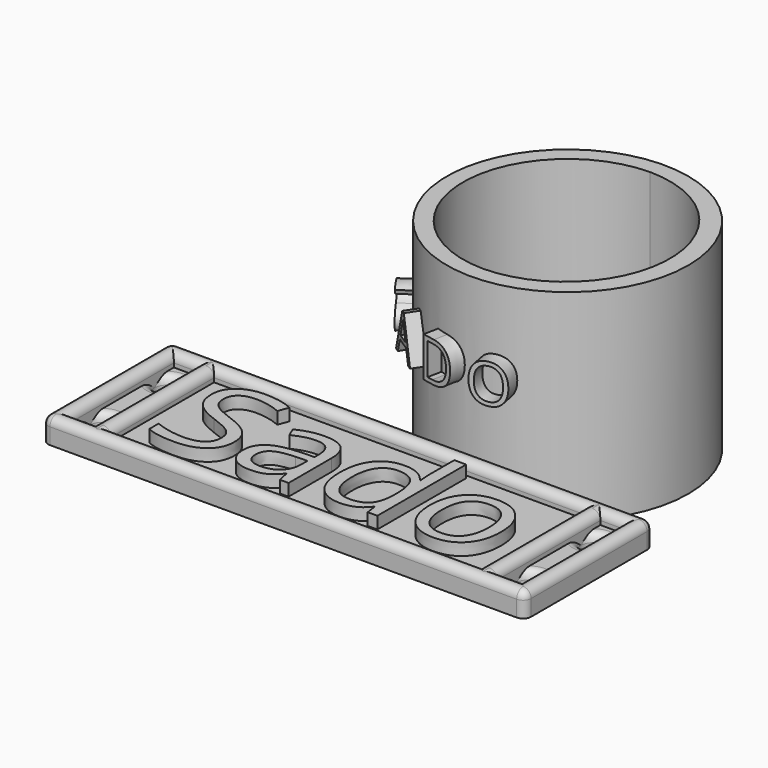
from build123d import *

# Parameters (mm, degrees)
F2_DEPTH       = 12.5
F3_TEXT_SIZE   = 7.2267029383
F4_DEPTH       = 2
F5_TEXT_SIZE   = 7.1017000462
F6_DEPTH       = 2
F7_TEXT_SIZE   = 6.9642465355
F8_DEPTH       = 2
F9_TEXT_SIZE   = 6.6435236173
F10_DEPTH      = 2
F1_R           = 15
F1_R_2         = 13
F11_DEPTH      = 12.5
F12_R          = 13
F13_DEPTH      = 70
F14_DEPTH      = 12.5
F15_W          = 46
F15_H          = 16
F15_TEXT_SIZE  = 18.1491124547
F16_DEPTH      = 3
F17_DEPTH      = 1.5
F18_T1_DEPTH   = 18
F18_T3_DEPTH   = 58
F18_T5_DEPTH   = 16
F18_T7_DEPTH   = 3
F18_T9_DEPTH   = 46
F18_T11_DEPTH  = 3
F18_T13_DEPTH  = 4.5
F18_S17_W      = 1.02
F18_S17_H      = 1.02
F18_T18_DEPTH  = 1.02
F18_S23_W      = 1.02
F18_S23_H      = 1.02
F18_T24_DEPTH  = 1.02
F18_S29_W      = 1.02
F18_S29_H      = 1.02
F18_T30_DEPTH  = 1.02
F18_S35_W      = 1.02
F18_S35_H      = 1.02
F18_T36_DEPTH  = 1.02
F18_T42_DEPTH  = 8
F18_T47_DEPTH  = 8
F18_T52_DEPTH  = 51
F18_T57_DEPTH  = 51
F18_T62_DEPTH  = 51
F18_T67_DEPTH  = 51
F18_T72_DEPTH  = 8
F18_T77_DEPTH  = 8
F18_T82_ANGLE  = 180
F18_T88_ANGLE  = 180
F18_T94_ANGLE  = 180
F18_T100_ANGLE = 180
F18_T106_ANGLE = 180
F18_T112_ANGLE = 180
F18_T118_ANGLE = 180
F18_T124_ANGLE = 180
F18_T131_DEPTH = 18.5
F18_T136_DEPTH = 5.5
F18_T144_DEPTH = 18.5
F18_T149_DEPTH = 5.5
F18_T157_DEPTH = 5.5
F18_T162_DEPTH = 18.5
F18_T170_DEPTH = 18.5
F18_T175_DEPTH = 5.5
F18_T183_DEPTH = 48.5
F18_T188_DEPTH = 18.5
F18_T196_DEPTH = 48.5
F18_T201_DEPTH = 18.5
F18_T209_DEPTH = 18.5
F18_T214_DEPTH = 48.5
F18_T222_DEPTH = 48.5
F18_T227_DEPTH = 18.5
F18_T235_DEPTH = 5.5
F18_T240_DEPTH = 18.5
F18_T248_DEPTH = 5.5
F18_T253_DEPTH = 18.5
F18_T261_DEPTH = 18.5
F18_T266_DEPTH = 5.5
F18_T274_DEPTH = 5.5
F18_T279_DEPTH = 18.5


# Not quite as in the source:
# - a fillet or chamfer that OpenCascade refuses, or shapes differently, is made with other operations: its cross-section is extruded or revolved along the edge and cut away or added
# - Text() gives the source's letters only with a copy of the font that has no kerning and outlines rounded to 1/6400 em; it was checked with that copy


with BuildPart() as f2:
    # F0 (on Top) → F2 (new body, symmetric)
    with BuildSketch(Plane.XY):
        Polygon((-5.7402514855, -13.8581929877), (0, -15), (5.7402514855, -13.8581929877), (10.6066017178, -10.6066017178), (13.8581929877, -5.7402514855), (15, 0), (13.8581929877, 5.7402514855), (10.6066017178, 10.6066017178), (5.7402514855, 13.8581929877), (0, 15), (-5.7402514855, 13.8581929877), (-10.6066017178, 10.6066017178), (-13.8581929877, 5.7402514855), (-15, 0), (-13.8581929877, -5.7402514855), (-10.6066017178, -10.6066017178), align=None)
    extrude(amount=F2_DEPTH, both=True)

    # F3 (on face) → F4 (join)
    with BuildSketch(Plane(origin=(-12.2323973527, -8.1734266016, 0), x_dir=(0.555570233, -0.8314696123, 0), z_dir=(-0.8314696123, -0.555570233, 0))):
        with Locations((-2.0443665109, 0)):
            Text('S', F3_TEXT_SIZE, font='Open Sans', text_align=(TextAlign.LEFT, TextAlign.BOTTOM))
    extrude(amount=F4_DEPTH)

    # F5 (on face) → F6 (join)
    with BuildSketch(Plane(origin=(-8.1734266016, -12.2323973527, 0), x_dir=(0.8314696123, -0.555570233, 0), z_dir=(-0.555570233, -0.8314696123, 0))):
        with Locations((-2.3712676484, 0)):
            Text('A', F5_TEXT_SIZE, font='Open Sans', text_align=(TextAlign.LEFT, TextAlign.BOTTOM))
    extrude(amount=F6_DEPTH)

    # F7 (on face) → F8 (join)
    with BuildSketch(Plane(origin=(-2.8701257427, -14.4290964938, 0), x_dir=(0.9807852804, -0.195090322, 0), z_dir=(-0.195090322, -0.9807852804, 0))):
        with Locations((-2.5102309883, 0)):
            Text('D', F7_TEXT_SIZE, font='Open Sans', text_align=(TextAlign.LEFT, TextAlign.BOTTOM))
    extrude(amount=F8_DEPTH)

    # F9 (on face) → F10 (join)
    with BuildSketch(Plane(origin=(2.8701257427, -14.4290964938, 0), x_dir=(0.9807852804, 0.195090322, 0), z_dir=(0.195090322, -0.9807852804, 0))):
        with Locations((-2.5762089062, 0)):
            Text('O', F9_TEXT_SIZE, font='Open Sans', text_align=(TextAlign.LEFT, TextAlign.BOTTOM))
    extrude(amount=F10_DEPTH)

    # F1 (on Top) → F11 (join, symmetric)
    with BuildSketch(Plane.XY):
        Circle(F1_R)
        Circle(F1_R_2, mode=Mode.SUBTRACT)
    extrude(amount=F11_DEPTH, both=True)

    # F12 (on face) → F13 (cut)
    with BuildSketch(Plane(origin=(0, 0, -12.5), x_dir=(1, 0, 0), z_dir=(0, 0, -1))):
        with Locations((-0.2790116705, 0)):
            Circle(F12_R)
    extrude(amount=-F13_DEPTH, mode=Mode.SUBTRACT)

    # F1 (on Top) → F14 (join, symmetric)
    with BuildSketch(Plane.XY):
        Circle(F1_R)
        Circle(F1_R_2, mode=Mode.SUBTRACT)
    extrude(amount=F14_DEPTH, both=True)


with BuildPart() as f16:
    # F15 (on Top) → F16 (new body)
    with BuildSketch(Plane.XY):
        Polygon((29.2240764946, -29.4431182742), (-20.7759235054, -29.4431182742), (-20.7759235054, -31.4431182742), (-20.7759235054, -34.4431193173), (-20.7759235054, -44.4431193173), (-20.7759235054, -47.4431182742), (-20.7759235054, -49.4431182742), (29.2240764946, -49.4431182742), (34.2240764946, -49.4431182742), (34.2240764946, -29.4431182742), align=None)
        with Locations((4.2240764946, -39.4431182742)):
            Rectangle(F15_W, F15_H, mode=Mode.SUBTRACT)
        Polygon((32.2240764946, -47.4431182742), (29.2240764946, -47.4431182742), (29.2240764946, -44.4431193173), (29.2240764946, -34.4431193173), (29.2240764946, -31.4431182742), (32.2240764946, -31.4431182742), (32.2240764946, -34.4431193173), (32.2240764946, -44.4431193173), align=None, mode=Mode.SUBTRACT)
        Polygon((-20.7759235054, -31.4431182742), (-20.7759235054, -29.4431182742), (-25.7759235054, -29.4431182742), (-25.7759235054, -49.4431182742), (-20.7759235054, -49.4431182742), (-20.7759235054, -47.4431182742), (-23.7759235054, -47.4431182742), (-23.7759235054, -44.4431193173), (-23.7759235054, -34.4431193173), (-23.7759235054, -31.4431182742), align=None)
        with Locations((-16.7070478201, -45.6872321665)):
            Text('Sado', F15_TEXT_SIZE, font='Open Sans', text_align=(TextAlign.LEFT, TextAlign.BOTTOM))
    extrude(amount=F16_DEPTH)

    # F15 (on Top) → F17 (join)
    with BuildSketch(Plane.XY):
        with Locations((4.2240764946, -39.4431182742)):
            Rectangle(F15_W, F15_H)
        with BuildLine():
            Line((1.8787776531, -45.6872321665), (0.786995107, -45.6872321665))
            Line((0.786995107, -45.6872321665), (0.4949078284, -44.3033623419))
            Line((0.4949078284, -44.3033623419), (0.4240128579, -44.3033623419))
            add(Edge.make_bspline(
                [(0.4240128579, -44.3033623419), (-0.3019516403, -45.2164895622), (-1.0236624403, -45.5411885272)],
                knots=[0, 0, 0, 1, 1, 1], degree=2))
            add(Edge.make_bspline(
                [(-1.0236624403, -45.5411885272), (-1.7453732402, -45.8658874923), (-2.8286483899, -45.8658874923)],
                knots=[0, 0, 0, 1, 1, 1], degree=2))
            add(Edge.make_bspline(
                [(-2.8286483899, -45.8658874923), (-4.2720699898, -45.8658874923), (-5.0916158491, -45.1200724023)],
                knots=[0, 0, 0, 1, 1, 1], degree=2))
            add(Edge.make_bspline(
                [(-5.0916158491, -45.1200724023), (-5.9111617084, -44.3742573124), (-5.9111617084, -43.001730683)],
                knots=[0, 0, 0, 1, 1, 1], degree=2))
            add(Edge.make_bspline(
                [(-5.9111617084, -43.001730683), (-5.9111617084, -40.0610073056), (-1.2065714642, -39.9192173645)],
                knots=[0, 0, 0, 1, 1, 1], degree=2))
            Line((-1.2065714642, -39.9192173645), (0.4410276508, -39.8653371869))
            Line((0.4410276508, -39.8653371869), (0.4410276508, -39.261312038))
            add(Edge.make_bspline(
                [(0.4410276508, -39.261312038), (0.4410276508, -38.1184851131), (-0.0495655452, -37.5740117395)],
                knots=[0, 0, 0, 1, 1, 1], degree=2))
            add(Edge.make_bspline(
                [(-0.0495655452, -37.5740117395), (-0.5401587413, -37.0295383659), (-1.6234338909, -37.0295383659)],
                knots=[0, 0, 0, 1, 1, 1], degree=2))
            add(Edge.make_bspline(
                [(-1.6234338909, -37.0295383659), (-2.8371557863, -37.0295383659), (-4.3684871497, -37.772517657)],
                knots=[0, 0, 0, 1, 1, 1], degree=2))
            Line((-4.3684871497, -37.772517657), (-4.8222149611, -36.646705525))
            add(Edge.make_bspline(
                [(-4.8222149611, -36.646705525), (-4.1047578593, -36.2582010865), (-3.2497645148, -36.0370087785)],
                knots=[0, 0, 0, 1, 1, 1], degree=2))
            add(Edge.make_bspline(
                [(-3.2497645148, -36.0370087785), (-2.3947711703, -35.8158164705), (-1.5326883287, -35.8158164705)],
                knots=[0, 0, 0, 1, 1, 1], degree=2))
            add(Edge.make_bspline(
                [(-1.5326883287, -35.8158164705), (0.2028205498, -35.8158164705), (1.0407991014, -36.5857358504)],
                knots=[0, 0, 0, 1, 1, 1], degree=2))
            add(Edge.make_bspline(
                [(1.0407991014, -36.5857358504), (1.8787776531, -37.3556552303), (1.8787776531, -39.0571345229)],
                knots=[0, 0, 0, 1, 1, 1], degree=2))
            Line((1.8787776531, -39.0571345229), (1.8787776531, -45.6872321665))
        make_face(mode=Mode.SUBTRACT)
        with BuildLine():
            add(Edge.make_bspline(
                [(23.2110742844, -37.1528956146), (24.4120350851, -38.5098253505), (24.4120350851, -40.8210013896)],
                knots=[0, 0, 0, 1, 1, 1], degree=2))
            add(Edge.make_bspline(
                [(24.4120350851, -40.8210013896), (24.4120350851, -43.1974008016), (23.2167458821, -44.531644147)],
                knots=[0, 0, 0, 1, 1, 1], degree=2))
            add(Edge.make_bspline(
                [(23.2167458821, -44.531644147), (22.021456679, -45.8658874923), (19.9116223561, -45.8658874923)],
                knots=[0, 0, 0, 1, 1, 1], degree=2))
            add(Edge.make_bspline(
                [(19.9116223561, -45.8658874923), (18.6071548984, -45.8658874923), (17.5976105181, -45.2533549469)],
                knots=[0, 0, 0, 1, 1, 1], degree=2))
            add(Edge.make_bspline(
                [(17.5976105181, -45.2533549469), (16.5880661379, -44.6408224016), (16.0379211666, -43.4979954767)],
                knots=[0, 0, 0, 1, 1, 1], degree=2))
            add(Edge.make_bspline(
                [(16.0379211666, -43.4979954767), (15.4877761953, -42.3551685518), (15.4877761953, -40.8210013896)],
                knots=[0, 0, 0, 1, 1, 1], degree=2))
            add(Edge.make_bspline(
                [(15.4877761953, -40.8210013896), (15.4877761953, -38.4474377764), (16.6759759013, -37.1217018275)],
                knots=[0, 0, 0, 1, 1, 1], degree=2))
            add(Edge.make_bspline(
                [(16.6759759013, -37.1217018275), (17.8641756073, -35.7959658787), (19.9740099302, -35.7959658787)],
                knots=[0, 0, 0, 1, 1, 1], degree=2))
            add(Edge.make_bspline(
                [(19.9740099302, -35.7959658787), (22.0101134837, -35.7959658787), (23.2110742844, -37.1528956146)],
                knots=[0, 0, 0, 1, 1, 1], degree=2))
        make_face(mode=Mode.SUBTRACT)
        with BuildLine():
            add(Edge.make_bspline(
                [(-8.3811424815, -40.0780220985), (-7.6154767998, -40.9117469519), (-7.6154767998, -42.2389008001)],
                knots=[0, 0, 0, 1, 1, 1], degree=2))
            add(Edge.make_bspline(
                [(-7.6154767998, -42.2389008001), (-7.6154767998, -43.9488874892), (-8.856138784, -44.9073874907)],
                knots=[0, 0, 0, 1, 1, 1], degree=2))
            add(Edge.make_bspline(
                [(-8.856138784, -44.9073874907), (-10.0968007682, -45.8658874923), (-12.223649884, -45.8658874923)],
                knots=[0, 0, 0, 1, 1, 1], degree=2))
            add(Edge.make_bspline(
                [(-12.223649884, -45.8658874923), (-14.5263185267, -45.8658874923), (-15.7683984103, -45.2703697398)],
                knots=[0, 0, 0, 1, 1, 1], degree=2))
            Line((-15.7683984103, -45.2703697398), (-15.7683984103, -43.8184407435))
            add(Edge.make_bspline(
                [(-15.7683984103, -43.8184407435), (-14.9687031428, -44.1530650043), (-14.030053733, -44.348735123)],
                knots=[0, 0, 0, 1, 1, 1], degree=2))
            add(Edge.make_bspline(
                [(-14.030053733, -44.348735123), (-13.0914043233, -44.5444052416), (-12.1697697064, -44.5444052416)],
                knots=[0, 0, 0, 1, 1, 1], degree=2))
            add(Edge.make_bspline(
                [(-12.1697697064, -44.5444052416), (-10.6639605324, -44.5444052416), (-9.9011306496, -43.9729917792)],
                knots=[0, 0, 0, 1, 1, 1], degree=2))
            add(Edge.make_bspline(
                [(-9.9011306496, -43.9729917792), (-9.1383007667, -43.4015783168), (-9.1383007667, -42.3806907412)],
                knots=[0, 0, 0, 1, 1, 1], degree=2))
            add(Edge.make_bspline(
                [(-9.1383007667, -42.3806907412), (-9.1383007667, -41.7086064206), (-9.4091195541, -41.2789828992)],
                knots=[0, 0, 0, 1, 1, 1], degree=2))
            add(Edge.make_bspline(
                [(-9.4091195541, -41.2789828992), (-9.6799383415, -40.8493593778), (-10.313739378, -40.4849592293)],
                knots=[0, 0, 0, 1, 1, 1], degree=2))
            add(Edge.make_bspline(
                [(-10.313739378, -40.4849592293), (-10.9475404145, -40.1205590808), (-12.2406646769, -39.6611596718)],
                knots=[0, 0, 0, 1, 1, 1], degree=2))
            add(Edge.make_bspline(
                [(-12.2406646769, -39.6611596718), (-14.0470685259, -39.0145975406), (-14.8226595035, -38.128410409)],
                knots=[0, 0, 0, 1, 1, 1], degree=2))
            add(Edge.make_bspline(
                [(-14.8226595035, -38.128410409), (-15.5982504811, -37.2422232774), (-15.5982504811, -35.8158164705)],
                knots=[0, 0, 0, 1, 1, 1], degree=2))
            add(Edge.make_bspline(
                [(-15.5982504811, -35.8158164705), (-15.5982504811, -34.3185146929), (-14.4738562485, -33.4323275614)],
                knots=[0, 0, 0, 1, 1, 1], degree=2))
            add(Edge.make_bspline(
                [(-14.4738562485, -33.4323275614), (-13.349462016, -32.5461404298), (-11.494849587, -32.5461404298)],
                knots=[0, 0, 0, 1, 1, 1], degree=2))
            add(Edge.make_bspline(
                [(-11.494849587, -32.5461404298), (-9.5636705899, -32.5461404298), (-7.9415936642, -33.255090135)],
                knots=[0, 0, 0, 1, 1, 1], degree=2))
            Line((-7.9415936642, -33.255090135), (-8.4123362685, -34.5652291904))
            add(Edge.make_bspline(
                [(-8.4123362685, -34.5652291904), (-10.0173984012, -33.8931448698), (-11.5317149717, -33.8931448698)],
                knots=[0, 0, 0, 1, 1, 1], degree=2))
            add(Edge.make_bspline(
                [(-11.5317149717, -33.8931448698), (-12.7284220742, -33.8931448698), (-13.4019242942, -34.4064244564)],
                knots=[0, 0, 0, 1, 1, 1], degree=2))
            add(Edge.make_bspline(
                [(-13.4019242942, -34.4064244564), (-14.0754265142, -34.919704043), (-14.0754265142, -35.8328312634)],
                knots=[0, 0, 0, 1, 1, 1], degree=2))
            add(Edge.make_bspline(
                [(-14.0754265142, -35.8328312634), (-14.0754265142, -36.504915584), (-13.8272941173, -36.9359570048)],
                knots=[0, 0, 0, 1, 1, 1], degree=2))
            add(Edge.make_bspline(
                [(-13.8272941173, -36.9359570048), (-13.5791617205, -37.3669984256), (-12.9893155657, -37.7257269764)],
                knots=[0, 0, 0, 1, 1, 1], degree=2))
            add(Edge.make_bspline(
                [(-12.9893155657, -37.7257269764), (-12.3994694109, -38.0844555273), (-11.1857475155, -38.5183327469)],
                knots=[0, 0, 0, 1, 1, 1], degree=2))
            add(Edge.make_bspline(
                [(-11.1857475155, -38.5183327469), (-9.1468081632, -39.2442972451), (-8.3811424815, -40.0780220985)],
                knots=[0, 0, 0, 1, 1, 1], degree=2))
        make_face(mode=Mode.SUBTRACT)
        with BuildLine():
            Line((11.7133279645, -45.6872321665), (11.5176578458, -44.3856005077))
            Line((11.5176578458, -44.3856005077), (11.4382554788, -44.3856005077))
            add(Edge.make_bspline(
                [(11.4382554788, -44.3856005077), (10.4202037021, -45.8658874923), (8.3897717462, -45.8658874923)],
                knots=[0, 0, 0, 1, 1, 1], degree=2))
            add(Edge.make_bspline(
                [(8.3897717462, -45.8658874923), (6.4841149385, -45.8658874923), (5.4249440788, -44.562837934)],
                knots=[0, 0, 0, 1, 1, 1], degree=2))
            add(Edge.make_bspline(
                [(5.4249440788, -44.562837934), (4.3657732191, -43.2597883757), (4.3657732191, -40.8578667743)],
                knots=[0, 0, 0, 1, 1, 1], degree=2))
            add(Edge.make_bspline(
                [(4.3657732191, -40.8578667743), (4.3657732191, -38.4559451729), (5.429197777, -37.1259555258)],
                knots=[0, 0, 0, 1, 1, 1], degree=2))
            add(Edge.make_bspline(
                [(5.429197777, -37.1259555258), (6.4926223349, -35.7959658787), (8.3897717462, -35.7959658787)],
                knots=[0, 0, 0, 1, 1, 1], degree=2))
            add(Edge.make_bspline(
                [(8.3897717462, -35.7959658787), (10.3663235245, -35.7959658787), (11.4212406859, -37.233715881)],
                knots=[0, 0, 0, 1, 1, 1], degree=2))
            Line((11.4212406859, -37.233715881), (11.5375084376, -37.233715881))
            Line((11.5375084376, -37.233715881), (11.4751208635, -36.5332735722))
            Line((11.4751208635, -36.5332735722), (11.4382554788, -35.8498460563))
            Line((11.4382554788, -35.8498460563), (11.4382554788, -31.8967424998))
            Line((11.4382554788, -31.8967424998), (12.910035067, -31.8967424998))
            Line((12.910035067, -31.8967424998), (12.910035067, -45.6872321665))
            Line((12.910035067, -45.6872321665), (11.7133279645, -45.6872321665))
        make_face(mode=Mode.SUBTRACT)
        with BuildLine():
            add(Edge.make_bspline(
                [(17.7493257551, -37.9951278644), (17.013435961, -38.9437025701), (17.013435961, -40.8210013896)],
                knots=[0, 0, 0, 1, 1, 1], degree=2))
            add(Edge.make_bspline(
                [(17.013435961, -40.8210013896), (17.013435961, -42.684121215), (17.7578331515, -43.6582181101)],
                knots=[0, 0, 0, 1, 1, 1], degree=2))
            add(Edge.make_bspline(
                [(17.7578331515, -43.6582181101), (18.5022303421, -44.6323150051), (19.945651942, -44.6323150051)],
                knots=[0, 0, 0, 1, 1, 1], degree=2))
            add(Edge.make_bspline(
                [(19.945651942, -44.6323150051), (21.3919093407, -44.6323150051), (22.1405602295, -43.6624718083)],
                knots=[0, 0, 0, 1, 1, 1], degree=2))
            add(Edge.make_bspline(
                [(22.1405602295, -43.6624718083), (22.8892111182, -42.6926286115), (22.8892111182, -40.8210013896)],
                knots=[0, 0, 0, 1, 1, 1], degree=2))
            add(Edge.make_bspline(
                [(22.8892111182, -40.8210013896), (22.8892111182, -38.9692247595), (22.1405602295, -38.0078889591)],
                knots=[0, 0, 0, 1, 1, 1], degree=2))
            add(Edge.make_bspline(
                [(22.1405602295, -38.0078889591), (21.3919093407, -37.0465531588), (19.9286371491, -37.0465531588)],
                knots=[0, 0, 0, 1, 1, 1], degree=2))
            add(Edge.make_bspline(
                [(19.9286371491, -37.0465531588), (18.4852155491, -37.0465531588), (17.7493257551, -37.9951278644)],
                knots=[0, 0, 0, 1, 1, 1], degree=2))
        make_face()
        with BuildLine():
            Line((29.2240764946, -34.4431193173), (29.2240764946, -44.4431193173))
            ThreePointArc((29.2240765542, -44.4431193173), (30.7240765542, -42.9431193173), (32.2240765542, -44.4431193173))
            Line((32.2240764946, -44.4431193173), (32.2240764946, -34.4431193173))
            ThreePointArc((32.2240765542, -34.4431193173), (30.7240765542, -35.9431193173), (29.2240765542, -34.4431193173))
        make_face()
        with BuildLine():
            Line((29.2240764946, -31.4431182742), (29.2240764946, -34.4431193173))
            ThreePointArc((29.2240765542, -34.4431193173), (30.7240765542, -32.9431193173), (32.2240765542, -34.4431193173))
            Line((32.2240764946, -34.4431193173), (32.2240764946, -31.4431182742))
            Line((32.2240764946, -31.4431182742), (29.2240764946, -31.4431182742))
        make_face()
        with BuildLine():
            Line((29.2240764946, -44.4431193173), (29.2240764946, -47.4431182742))
            Line((29.2240764946, -47.4431182742), (32.2240764946, -47.4431182742))
            Line((32.2240764946, -47.4431182742), (32.2240764946, -44.4431193173))
            ThreePointArc((32.2240765542, -44.4431193173), (30.7240765542, -45.9431193173), (29.2240765542, -44.4431193173))
        make_face()
        with BuildLine():
            add(Edge.make_bspline(
                [(6.5734426013, -43.6837402995), (7.2554522178, -44.6323150051), (8.5769344684, -44.6323150051)],
                knots=[0, 0, 0, 1, 1, 1], degree=2))
            add(Edge.make_bspline(
                [(8.5769344684, -44.6323150051), (10.0827436424, -44.6323150051), (10.7604995606, -43.8127691458)],
                knots=[0, 0, 0, 1, 1, 1], degree=2))
            add(Edge.make_bspline(
                [(10.7604995606, -43.8127691458), (11.4382554788, -42.9932232865), (11.4382554788, -41.1669688458)],
                knots=[0, 0, 0, 1, 1, 1], degree=2))
            Line((11.4382554788, -41.1669688458), (11.4382554788, -40.8578667743))
            add(Edge.make_bspline(
                [(11.4382554788, -40.8578667743), (11.4382554788, -38.7934052326), (10.7519921641, -37.9114717992)],
                knots=[0, 0, 0, 1, 1, 1], degree=2))
            add(Edge.make_bspline(
                [(10.7519921641, -37.9114717992), (10.0657288494, -37.0295383659), (8.5599196755, -37.0295383659)],
                knots=[0, 0, 0, 1, 1, 1], degree=2))
            add(Edge.make_bspline(
                [(8.5599196755, -37.0295383659), (7.2639596142, -37.0295383659), (6.5776962995, -38.0348290479)],
                knots=[0, 0, 0, 1, 1, 1], degree=2))
            add(Edge.make_bspline(
                [(6.5776962995, -38.0348290479), (5.8914329849, -39.04011973), (5.8914329849, -40.8748815672)],
                knots=[0, 0, 0, 1, 1, 1], degree=2))
            add(Edge.make_bspline(
                [(5.8914329849, -40.8748815672), (5.8914329849, -42.7351655938), (6.5734426013, -43.6837402995)],
                knots=[0, 0, 0, 1, 1, 1], degree=2))
        make_face()
        with BuildLine():
            add(Edge.make_bspline(
                [(-3.8864013501, -44.2338852707), (-3.4043155505, -44.649329798), (-2.5365611113, -44.649329798)],
                knots=[0, 0, 0, 1, 1, 1], degree=2))
            add(Edge.make_bspline(
                [(-2.5365611113, -44.649329798), (-1.1611986831, -44.649329798), (-0.3771003091, -43.896425211)],
                knots=[0, 0, 0, 1, 1, 1], degree=2))
            add(Edge.make_bspline(
                [(-0.3771003091, -43.896425211), (0.4069980649, -43.143520624), (0.4069980649, -41.7880087876)],
                knots=[0, 0, 0, 1, 1, 1], degree=2))
            Line((0.4069980649, -41.7880087876), (0.4069980649, -40.9117469519))
            Line((0.4069980649, -40.9117469519), (-1.0647815232, -40.9712987271))
            add(Edge.make_bspline(
                [(-1.0647815232, -40.9712987271), (-2.8201409934, -41.0336863012), (-3.5943140716, -41.5171900002)],
                knots=[0, 0, 0, 1, 1, 1], degree=2))
            add(Edge.make_bspline(
                [(-3.5943140716, -41.5171900002), (-4.3684871497, -42.0006936992), (-4.3684871497, -43.0187454759)],
                knots=[0, 0, 0, 1, 1, 1], degree=2))
            add(Edge.make_bspline(
                [(-4.3684871497, -43.0187454759), (-4.3684871497, -43.8184407435), (-3.8864013501, -44.2338852707)],
                knots=[0, 0, 0, 1, 1, 1], degree=2))
        make_face()
        with BuildLine():
            Line((-20.7759235054, -44.4431193173), (-20.7759235054, -34.4431193173))
            ThreePointArc((-20.775923565, -34.4431193173), (-22.275923565, -35.9431193173), (-23.775923565, -34.4431193173))
            Line((-23.7759235054, -34.4431193173), (-23.7759235054, -44.4431193173))
            ThreePointArc((-23.775923565, -44.4431193173), (-22.275923565, -42.9431193173), (-20.775923565, -44.4431193173))
        make_face()
        with BuildLine():
            Line((-20.7759235054, -34.4431193173), (-20.7759235054, -31.4431182742))
            Line((-20.7759235054, -31.4431182742), (-23.7759235054, -31.4431182742))
            Line((-23.7759235054, -31.4431182742), (-23.7759235054, -34.4431193173))
            ThreePointArc((-23.775923565, -34.4431193173), (-22.275923565, -32.9431193173), (-20.775923565, -34.4431193173))
        make_face()
        with BuildLine():
            Line((-20.7759235054, -47.4431182742), (-20.7759235054, -44.4431193173))
            ThreePointArc((-20.775923565, -44.4431193173), (-22.275923565, -45.9431193173), (-23.775923565, -44.4431193173))
            Line((-23.7759235054, -44.4431193173), (-23.7759235054, -47.4431182742))
            Line((-23.7759235054, -47.4431182742), (-20.7759235054, -47.4431182742))
        make_face()
    extrude(amount=F17_DEPTH)

    # F18: fillet of radius 1 on 28 edges, made by hand

    # F18_s2 → F18_t1 (cut)
    with BuildSketch(Plane.XZ.offset(30.4431182742)):
        with BuildLine():
            ThreePointArc((-25.7759235054, 2), (-25.4830302866, 2.7071067812), (-24.7759235054, 3))
            Line((-24.7759235054, 3), (-25.7759235054, 3))
            Line((-25.7759235054, 3), (-25.7759235054, 2))
        make_face()
        with BuildLine():
            ThreePointArc((33.2240764946, 3), (33.9311832758, 2.7071067812), (34.2240764946, 2))
            Line((34.2240764946, 2), (34.2240764946, 3))
            Line((34.2240764946, 3), (33.2240764946, 3))
        make_face()
    extrude(amount=F18_T1_DEPTH, mode=Mode.SUBTRACT)

    # F18_s4 → F18_t3 (cut)
    with BuildSketch(Plane.YZ.offset(-24.7759235054)):
        with BuildLine():
            ThreePointArc((-48.4431182742, 3), (-49.1502250554, 2.7071067812), (-49.4431182742, 2))
            Line((-49.4431182742, 2), (-49.4431182742, 3))
            Line((-49.4431182742, 3), (-48.4431182742, 3))
        make_face()
        with BuildLine():
            ThreePointArc((-30.4431182742, 3), (-29.736011493, 2.7071067812), (-29.4431182742, 2))
            Line((-29.4431182742, 2), (-29.4431182742, 3))
            Line((-29.4431182742, 3), (-30.4431182742, 3))
        make_face()
    extrude(amount=F18_T3_DEPTH, mode=Mode.SUBTRACT)

    # F18_s6 → F18_t5 (cut)
    with BuildSketch(Plane.XZ.offset(31.4431182742)):
        with BuildLine():
            ThreePointArc((-19.7759235054, 3), (-20.4830302866, 2.7071067812), (-20.7759235054, 2))
            Line((-20.7759235054, 2), (-20.7759235054, 3))
            Line((-20.7759235054, 3), (-19.7759235054, 3))
        make_face()
        with BuildLine():
            ThreePointArc((-24.7759235054, 3), (-24.0688167242, 2.7071067812), (-23.7759235054, 2))
            Line((-23.7759235054, 2), (-23.7759235054, 3))
            Line((-23.7759235054, 3), (-24.7759235054, 3))
        make_face()
        with BuildLine():
            ThreePointArc((-19.7759235054, 3), (-19.0688167242, 2.7071067812), (-18.7759235054, 2))
            Line((-18.7759235054, 2), (-18.7759235054, 3))
            Line((-18.7759235054, 3), (-19.7759235054, 3))
        make_face()
        with BuildLine():
            ThreePointArc((28.2240764946, 3), (27.5169697134, 2.7071067812), (27.2240764946, 2))
            Line((27.2240764946, 2), (27.2240764946, 3))
            Line((27.2240764946, 3), (28.2240764946, 3))
        make_face()
        with BuildLine():
            ThreePointArc((33.2240764946, 3), (32.5169697134, 2.7071067812), (32.2240764946, 2))
            Line((32.2240764946, 2), (32.2240764946, 3))
            Line((32.2240764946, 3), (33.2240764946, 3))
        make_face()
        with BuildLine():
            ThreePointArc((28.2240764946, 3), (28.9311832758, 2.7071067812), (29.2240764946, 2))
            Line((29.2240764946, 2), (29.2240764946, 3))
            Line((29.2240764946, 3), (28.2240764946, 3))
        make_face()
    extrude(amount=F18_T5_DEPTH, mode=Mode.SUBTRACT)

    # F18_s8 → F18_t7 (cut)
    with BuildSketch(Plane.YZ.offset(-23.7759235054)):
        with BuildLine():
            ThreePointArc((-48.4431182742, 3), (-47.736011493, 2.7071067812), (-47.4431182742, 2))
            Line((-47.4431182742, 2), (-47.4431182742, 3))
            Line((-47.4431182742, 3), (-48.4431182742, 3))
        make_face()
        with BuildLine():
            ThreePointArc((-30.4431182742, 3), (-31.1502250554, 2.7071067812), (-31.4431182742, 2))
            Line((-31.4431182742, 2), (-31.4431182742, 3))
            Line((-31.4431182742, 3), (-30.4431182742, 3))
        make_face()
    extrude(amount=F18_T7_DEPTH, mode=Mode.SUBTRACT)

    # F18_s10 → F18_t9 (cut)
    with BuildSketch(Plane.YZ.offset(-18.7759235054)):
        with BuildLine():
            ThreePointArc((-48.4431182742, 3), (-47.736011493, 2.7071067812), (-47.4431182742, 2))
            Line((-47.4431182742, 2), (-47.4431182742, 3))
            Line((-47.4431182742, 3), (-48.4431182742, 3))
        make_face()
        with BuildLine():
            ThreePointArc((-30.4431182742, 3), (-31.1502250554, 2.7071067812), (-31.4431182742, 2))
            Line((-31.4431182742, 2), (-31.4431182742, 3))
            Line((-31.4431182742, 3), (-30.4431182742, 3))
        make_face()
    extrude(amount=F18_T9_DEPTH, mode=Mode.SUBTRACT)

    # F18_s12 → F18_t11 (cut)
    with BuildSketch(Plane.YZ.offset(29.2240764946)):
        with BuildLine():
            ThreePointArc((-30.4431182742, 3), (-31.1502250554, 2.7071067812), (-31.4431182742, 2))
            Line((-31.4431182742, 2), (-31.4431182742, 3))
            Line((-31.4431182742, 3), (-30.4431182742, 3))
        make_face()
        with BuildLine():
            ThreePointArc((-48.4431182742, 3), (-47.736011493, 2.7071067812), (-47.4431182742, 2))
            Line((-47.4431182742, 2), (-47.4431182742, 3))
            Line((-47.4431182742, 3), (-48.4431182742, 3))
        make_face()
    extrude(amount=F18_T11_DEPTH, mode=Mode.SUBTRACT)

    # F18_s14 → F18_t13 (cut)
    with BuildSketch(Plane.XY.offset(-2.5)):
        with BuildLine():
            ThreePointArc((-25.7759235054, -48.4431182742), (-25.4830302866, -49.1502250554), (-24.7759235054, -49.4431182742))
            Line((-24.7759235054, -49.4431182742), (-25.7759235054, -49.4431182742))
            Line((-25.7759235054, -49.4431182742), (-25.7759235054, -48.4431182742))
        make_face()
        with BuildLine():
            ThreePointArc((-25.7759235054, -30.4431182742), (-25.4830302866, -29.736011493), (-24.7759235054, -29.4431182742))
            Line((-24.7759235054, -29.4431182742), (-25.7759235054, -29.4431182742))
            Line((-25.7759235054, -29.4431182742), (-25.7759235054, -30.4431182742))
        make_face()
        with BuildLine():
            ThreePointArc((34.2240764946, -30.4431182742), (33.9311832758, -29.736011493), (33.2240764946, -29.4431182742))
            Line((33.2240764946, -29.4431182742), (34.2240764946, -29.4431182742))
            Line((34.2240764946, -29.4431182742), (34.2240764946, -30.4431182742))
        make_face()
        with BuildLine():
            ThreePointArc((34.2240764946, -48.4431182742), (33.9311832758, -49.1502250554), (33.2240764946, -49.4431182742))
            Line((33.2240764946, -49.4431182742), (34.2240764946, -49.4431182742))
            Line((34.2240764946, -49.4431182742), (34.2240764946, -48.4431182742))
        make_face()
    extrude(amount=F18_T13_DEPTH, mode=Mode.SUBTRACT)


with BuildPart() as f18_tool16:
    # F18_s17 → F18_t18 (new body)
    with BuildSketch(Plane.YZ.offset(-24.7759235054)):
        with Locations((-29.9331182742, 2.51)):
            Rectangle(F18_S17_W, F18_S17_H)
    extrude(amount=-F18_T18_DEPTH)

    # F18_s19 → F18_t20 (revolve, cut)
    with BuildSketch(Plane(origin=(-24.7759235054, -30.4431182742, 2), x_dir=(0, -0.7071067812, -0.7071067812), z_dir=(0, 0.7071067812, -0.7071067812))):
        with BuildLine():
            ThreePointArc((0, -1), (1, 0), (0, 1))
            Line((0, 1), (0, -1))
        make_face()
    revolve(axis=Axis((-24.7759235054, -30.4431182742, 2), (-1, 0, 0)), mode=Mode.SUBTRACT)


with BuildPart() as f16_1:
    add(f16.part)

    # F18_t15: cut F18_tool16
    add(f18_tool16.part, mode=Mode.SUBTRACT)


with BuildPart() as f18_tool22:
    # F18_s23 → F18_t24 (new body)
    with BuildSketch(Plane.YZ.offset(-24.7759235054)):
        with Locations((-48.9531182742, 2.51)):
            Rectangle(F18_S23_W, F18_S23_H)
    extrude(amount=-F18_T24_DEPTH)

    # F18_s25 → F18_t26 (revolve, cut)
    with BuildSketch(Plane(origin=(-24.7759235054, -48.4431182742, 2), x_dir=(0, 0.7071067812, -0.7071067812), z_dir=(0, 0.7071067812, 0.7071067812))):
        with BuildLine():
            ThreePointArc((0, -1), (1, 0), (0, 1))
            Line((0, 1), (0, -1))
        make_face()
    revolve(axis=Axis((-24.7759235054, -48.4431182742, 2), (-1, 0, 0)), mode=Mode.SUBTRACT)


with BuildPart() as f16_2:
    add(f16_1.part)

    # F18_t21: cut F18_tool22
    add(f18_tool22.part, mode=Mode.SUBTRACT)


with BuildPart() as f18_tool28:
    # F18_s29 → F18_t30 (new body)
    with BuildSketch(Plane.YZ.offset(33.2240764946)):
        with Locations((-48.9531182742, 2.51)):
            Rectangle(F18_S29_W, F18_S29_H)
    extrude(amount=F18_T30_DEPTH)

    # F18_s31 → F18_t32 (revolve, cut)
    with BuildSketch(Plane(origin=(33.2240764946, -48.4431182742, 2), x_dir=(0, 0.7071067812, -0.7071067812), z_dir=(0, -0.7071067812, -0.7071067812))):
        with BuildLine():
            ThreePointArc((0, -1), (1, 0), (0, 1))
            Line((0, 1), (0, -1))
        make_face()
    revolve(axis=Axis((33.2240764946, -48.4431182742, 2), (1, 0, 0)), mode=Mode.SUBTRACT)


with BuildPart() as f16_3:
    add(f16_2.part)

    # F18_t27: cut F18_tool28
    add(f18_tool28.part, mode=Mode.SUBTRACT)


with BuildPart() as f18_tool34:
    # F18_s35 → F18_t36 (new body)
    with BuildSketch(Plane.YZ.offset(33.2240764946)):
        with Locations((-29.9331182742, 2.51)):
            Rectangle(F18_S35_W, F18_S35_H)
    extrude(amount=F18_T36_DEPTH)

    # F18_s37 → F18_t38 (revolve, cut)
    with BuildSketch(Plane(origin=(33.2240764946, -30.4431182742, 2), x_dir=(0, -0.7071067812, -0.7071067812), z_dir=(0, -0.7071067812, 0.7071067812))):
        with BuildLine():
            ThreePointArc((0, -1), (1, 0), (0, 1))
            Line((0, 1), (0, -1))
        make_face()
    revolve(axis=Axis((33.2240764946, -30.4431182742, 2), (1, 0, 0)), mode=Mode.SUBTRACT)


with BuildPart() as f16_4:
    add(f16_3.part)

    # F18_t33: cut F18_tool34
    add(f18_tool34.part, mode=Mode.SUBTRACT)


with BuildPart() as f18_tool40:
    # F18_s41 → F18_t42 (new body)
    with BuildSketch(Plane.YZ.offset(-18.2759235054)):
        with BuildLine():
            ThreePointArc((-48.4431182742, 3), (-47.736011493, 2.7071067812), (-47.4431182742, 2))
            Line((-47.4431182742, 2), (-47.4431182742, 3))
            Line((-47.4431182742, 3), (-48.4431182742, 3))
        make_face()
    extrude(amount=-F18_T42_DEPTH)

    split(bisect_by=Plane.YZ.offset(-18.7759235054), keep=Keep.TOP)


with BuildPart() as f16_5:
    add(f16_4.part)

    # F18_t39: cut F18_tool40
    add(f18_tool40.part, mode=Mode.SUBTRACT)


with BuildPart() as f18_tool45:
    # F18_s46 → F18_t47 (new body)
    with BuildSketch(Plane.YZ.offset(-26.2759235054)):
        with BuildLine():
            ThreePointArc((-30.4431182742, 3), (-31.1502250554, 2.7071067812), (-31.4431182742, 2))
            Line((-31.4431182742, 2), (-31.4431182742, 3))
            Line((-31.4431182742, 3), (-30.4431182742, 3))
        make_face()
    extrude(amount=F18_T47_DEPTH)

    split(bisect_by=Plane.YZ.offset(-18.7759235054), keep=Keep.TOP)


with BuildPart() as f16_6:
    add(f16_5.part)

    # F18_t44: cut F18_tool45
    add(f18_tool45.part, mode=Mode.SUBTRACT)


with BuildPart() as f18_tool50:
    # F18_s51 → F18_t52 (new body)
    with BuildSketch(Plane.YZ.offset(29.7240764946)):
        with BuildLine():
            ThreePointArc((-48.4431182742, 3), (-47.736011493, 2.7071067812), (-47.4431182742, 2))
            Line((-47.4431182742, 2), (-47.4431182742, 3))
            Line((-47.4431182742, 3), (-48.4431182742, 3))
        make_face()
    extrude(amount=-F18_T52_DEPTH)

    split(bisect_by=Plane.YZ.offset(29.2240764946), keep=Keep.TOP)


with BuildPart() as f16_7:
    add(f16_6.part)

    # F18_t49: cut F18_tool50
    add(f18_tool50.part, mode=Mode.SUBTRACT)


with BuildPart() as f18_tool55:
    # F18_s56 → F18_t57 (new body)
    with BuildSketch(Plane.YZ.offset(29.7240764946)):
        with BuildLine():
            ThreePointArc((-48.4431182742, 3), (-47.736011493, 2.7071067812), (-47.4431182742, 2))
            Line((-47.4431182742, 2), (-47.4431182742, 3))
            Line((-47.4431182742, 3), (-48.4431182742, 3))
        make_face()
    extrude(amount=-F18_T57_DEPTH)

    split(bisect_by=Plane.YZ.offset(-20.7759235054), keep=Keep.BOTTOM)


with BuildPart() as f16_8:
    add(f16_7.part)

    # F18_t54: cut F18_tool55
    add(f18_tool55.part, mode=Mode.SUBTRACT)


with BuildPart() as f18_tool60:
    # F18_s61 → F18_t62 (new body)
    with BuildSketch(Plane.YZ.offset(-21.2759235054)):
        with BuildLine():
            ThreePointArc((-30.4431182742, 3), (-31.1502250554, 2.7071067812), (-31.4431182742, 2))
            Line((-31.4431182742, 2), (-31.4431182742, 3))
            Line((-31.4431182742, 3), (-30.4431182742, 3))
        make_face()
    extrude(amount=F18_T62_DEPTH)

    split(bisect_by=Plane.YZ.offset(-20.7759235054), keep=Keep.BOTTOM)


with BuildPart() as f16_9:
    add(f16_8.part)

    # F18_t59: cut F18_tool60
    add(f18_tool60.part, mode=Mode.SUBTRACT)


with BuildPart() as f18_tool65:
    # F18_s66 → F18_t67 (new body)
    with BuildSketch(Plane.YZ.offset(-21.2759235054)):
        with BuildLine():
            ThreePointArc((-30.4431182742, 3), (-31.1502250554, 2.7071067812), (-31.4431182742, 2))
            Line((-31.4431182742, 2), (-31.4431182742, 3))
            Line((-31.4431182742, 3), (-30.4431182742, 3))
        make_face()
    extrude(amount=F18_T67_DEPTH)

    split(bisect_by=Plane.YZ.offset(29.2240764946), keep=Keep.TOP)


with BuildPart() as f16_10:
    add(f16_9.part)

    # F18_t64: cut F18_tool65
    add(f18_tool65.part, mode=Mode.SUBTRACT)


with BuildPart() as f18_tool70:
    # F18_s71 → F18_t72 (new body)
    with BuildSketch(Plane.YZ.offset(26.7240764946)):
        with BuildLine():
            ThreePointArc((-30.4431182742, 3), (-31.1502250554, 2.7071067812), (-31.4431182742, 2))
            Line((-31.4431182742, 2), (-31.4431182742, 3))
            Line((-31.4431182742, 3), (-30.4431182742, 3))
        make_face()
    extrude(amount=F18_T72_DEPTH)

    split(bisect_by=Plane.YZ.offset(27.2240764946), keep=Keep.BOTTOM)


with BuildPart() as f16_11:
    add(f16_10.part)

    # F18_t69: cut F18_tool70
    add(f18_tool70.part, mode=Mode.SUBTRACT)


with BuildPart() as f18_tool75:
    # F18_s76 → F18_t77 (new body)
    with BuildSketch(Plane.YZ.offset(34.7240764946)):
        with BuildLine():
            ThreePointArc((-48.4431182742, 3), (-47.736011493, 2.7071067812), (-47.4431182742, 2))
            Line((-47.4431182742, 2), (-47.4431182742, 3))
            Line((-47.4431182742, 3), (-48.4431182742, 3))
        make_face()
    extrude(amount=-F18_T77_DEPTH)

    split(bisect_by=Plane.YZ.offset(27.2240764946), keep=Keep.BOTTOM)


with BuildPart() as f16_12:
    add(f16_11.part)

    # F18_t74: cut F18_tool75
    add(f18_tool75.part, mode=Mode.SUBTRACT)


with BuildPart() as f18_tool80:
    # F18_s81 → F18_t82 (revolve)
    with BuildSketch(Plane.XZ.offset(44.4431193173)):
        with BuildLine():
            ThreePointArc((28.2240765542, 1.5), (28.9311833354, 1.2071067812), (29.2240765542, 0.5))
            Line((29.2240765542, 0.5), (29.2240765542, 1.5))
            Line((29.2240765542, 1.5), (28.2240765542, 1.5))
        make_face()
    revolve(axis=Axis((30.7240765542, -44.4431193173, 1.5), (0, 0, -1)), revolution_arc=F18_T82_ANGLE)

    split(bisect_by=Plane.YZ.offset(29.2240764946), keep=Keep.TOP)

    split(bisect_by=Plane.YZ.offset(32.2240764946), keep=Keep.BOTTOM)


with BuildPart() as f16_13:
    add(f16_12.part)

    # F18_t79: cut F18_tool80
    add(f18_tool80.part, mode=Mode.SUBTRACT)


with BuildPart() as f18_tool86:
    # F18_s87 → F18_t88 (revolve)
    with BuildSketch(Plane.XZ.offset(34.4431193173)):
        with BuildLine():
            ThreePointArc((32.2240765542, 0.5), (32.516969773, 1.2071067812), (33.2240765542, 1.5))
            Line((33.2240765542, 1.5), (32.2240765542, 1.5))
            Line((32.2240765542, 1.5), (32.2240765542, 0.5))
        make_face()
    revolve(axis=Axis((30.7240765542, -34.4431193173, 1.5), (0, 0, -1)), revolution_arc=F18_T88_ANGLE)

    split(bisect_by=Plane.YZ.offset(29.2240764946), keep=Keep.TOP)

    split(bisect_by=Plane.YZ.offset(32.2240764946), keep=Keep.BOTTOM)


with BuildPart() as f16_14:
    add(f16_13.part)

    # F18_t85: cut F18_tool86
    add(f18_tool86.part, mode=Mode.SUBTRACT)


with BuildPart() as f18_tool92:
    # F18_s93 → F18_t94 (revolve)
    with BuildSketch(Plane.XZ.offset(34.4431193173)):
        with BuildLine():
            ThreePointArc((28.2240765542, 1.5), (28.9311833354, 1.2071067812), (29.2240765542, 0.5))
            Line((29.2240765542, 0.5), (29.2240765542, 1.5))
            Line((29.2240765542, 1.5), (28.2240765542, 1.5))
        make_face()
    revolve(axis=Axis((30.7240765542, -34.4431193173, 1.5), (0, 0, -1)), revolution_arc=F18_T94_ANGLE)

    split(bisect_by=Plane.YZ.offset(29.2240764946), keep=Keep.TOP)

    split(bisect_by=Plane.YZ.offset(32.2240764946), keep=Keep.BOTTOM)


with BuildPart() as f16_15:
    add(f16_14.part)

    # F18_t91: cut F18_tool92
    add(f18_tool92.part, mode=Mode.SUBTRACT)


with BuildPart() as f18_tool98:
    # F18_s99 → F18_t100 (revolve)
    with BuildSketch(Plane.XZ.offset(44.4431193173)):
        with BuildLine():
            ThreePointArc((32.2240765542, 0.5), (32.516969773, 1.2071067812), (33.2240765542, 1.5))
            Line((33.2240765542, 1.5), (32.2240765542, 1.5))
            Line((32.2240765542, 1.5), (32.2240765542, 0.5))
        make_face()
    revolve(axis=Axis((30.7240765542, -44.4431193173, 1.5), (0, 0, -1)), revolution_arc=F18_T100_ANGLE)

    split(bisect_by=Plane.YZ.offset(29.2240764946), keep=Keep.TOP)

    split(bisect_by=Plane.YZ.offset(32.2240764946), keep=Keep.BOTTOM)


with BuildPart() as f16_16:
    add(f16_15.part)

    # F18_t97: cut F18_tool98
    add(f18_tool98.part, mode=Mode.SUBTRACT)


with BuildPart() as f18_tool104:
    # F18_s105 → F18_t106 (revolve)
    with BuildSketch(Plane.XZ.offset(34.4431193173)):
        with BuildLine():
            ThreePointArc((-20.775923565, 0.5), (-20.4830303462, 1.2071067812), (-19.775923565, 1.5))
            Line((-19.775923565, 1.5), (-20.775923565, 1.5))
            Line((-20.775923565, 1.5), (-20.775923565, 0.5))
        make_face()
    revolve(axis=Axis((-22.275923565, -34.4431193173, 1.5), (0, 0, -1)), revolution_arc=F18_T106_ANGLE)

    split(bisect_by=Plane.YZ.offset(-23.7759235054), keep=Keep.TOP)

    split(bisect_by=Plane.YZ.offset(-20.7759235054), keep=Keep.BOTTOM)


with BuildPart() as f16_17:
    add(f16_16.part)

    # F18_t103: cut F18_tool104
    add(f18_tool104.part, mode=Mode.SUBTRACT)


with BuildPart() as f18_tool110:
    # F18_s111 → F18_t112 (revolve)
    with BuildSketch(Plane.XZ.offset(34.4431193173)):
        with BuildLine():
            ThreePointArc((-24.775923565, 1.5), (-24.0688167838, 1.2071067812), (-23.775923565, 0.5))
            Line((-23.775923565, 0.5), (-23.775923565, 1.5))
            Line((-23.775923565, 1.5), (-24.775923565, 1.5))
        make_face()
    revolve(axis=Axis((-22.275923565, -34.4431193173, 1.5), (0, 0, -1)), revolution_arc=F18_T112_ANGLE)

    split(bisect_by=Plane.YZ.offset(-23.7759235054), keep=Keep.TOP)

    split(bisect_by=Plane.YZ.offset(-20.7759235054), keep=Keep.BOTTOM)


with BuildPart() as f16_18:
    add(f16_17.part)

    # F18_t109: cut F18_tool110
    add(f18_tool110.part, mode=Mode.SUBTRACT)


with BuildPart() as f18_tool116:
    # F18_s117 → F18_t118 (revolve)
    with BuildSketch(Plane.XZ.offset(44.4431193173)):
        with BuildLine():
            ThreePointArc((-24.775923565, 1.5), (-24.0688167838, 1.2071067812), (-23.775923565, 0.5))
            Line((-23.775923565, 0.5), (-23.775923565, 1.5))
            Line((-23.775923565, 1.5), (-24.775923565, 1.5))
        make_face()
    revolve(axis=Axis((-22.275923565, -44.4431193173, 1.5), (0, 0, -1)), revolution_arc=F18_T118_ANGLE)

    split(bisect_by=Plane.YZ.offset(-23.7759235054), keep=Keep.TOP)

    split(bisect_by=Plane.YZ.offset(-20.7759235054), keep=Keep.BOTTOM)


with BuildPart() as f16_19:
    add(f16_18.part)

    # F18_t115: cut F18_tool116
    add(f18_tool116.part, mode=Mode.SUBTRACT)


with BuildPart() as f18_tool122:
    # F18_s123 → F18_t124 (revolve)
    with BuildSketch(Plane.XZ.offset(44.4431193173)):
        with BuildLine():
            ThreePointArc((-20.775923565, 0.5), (-20.4830303462, 1.2071067812), (-19.775923565, 1.5))
            Line((-19.775923565, 1.5), (-20.775923565, 1.5))
            Line((-20.775923565, 1.5), (-20.775923565, 0.5))
        make_face()
    revolve(axis=Axis((-22.275923565, -44.4431193173, 1.5), (0, 0, -1)), revolution_arc=F18_T124_ANGLE)

    split(bisect_by=Plane.YZ.offset(-23.7759235054), keep=Keep.TOP)

    split(bisect_by=Plane.YZ.offset(-20.7759235054), keep=Keep.BOTTOM)


with BuildPart() as f16_20:
    add(f16_19.part)

    # F18_t121: cut F18_tool122
    add(f18_tool122.part, mode=Mode.SUBTRACT)


with BuildPart() as f18_tool129:
    # F18_s130 → F18_t131 (new body)
    with BuildSketch(Plane.XZ.offset(28.9431182742)):
        with BuildLine():
            ThreePointArc((-19.7759235054, 3), (-20.4830302866, 2.7071067812), (-20.7759235054, 2))
            Line((-20.7759235054, 2), (-20.7759235054, 3))
            Line((-20.7759235054, 3), (-19.7759235054, 3))
        make_face()
    extrude(amount=F18_T131_DEPTH)

    split(bisect_by=Plane.XZ.offset(31.4431182742), keep=Keep.BOTTOM)

    split(bisect_by=Plane.XZ.offset(29.4431182742), keep=Keep.TOP)


with BuildPart() as f18_tool134:
    # F18_s135 → F18_t136 (new body)
    with BuildSketch(Plane.YZ.offset(-23.7759235054)):
        with BuildLine():
            ThreePointArc((-30.4431182742, 3), (-31.1502250554, 2.7071067812), (-31.4431182742, 2))
            Line((-31.4431182742, 2), (-31.4431182742, 3))
            Line((-31.4431182742, 3), (-30.4431182742, 3))
        make_face()
    extrude(amount=F18_T136_DEPTH)

    split(bisect_by=Plane.YZ.offset(-18.7759235054), keep=Keep.BOTTOM)

    split(bisect_by=Plane.YZ.offset(-20.7759235054), keep=Keep.TOP)


with BuildPart() as f18_tool129_1:
    add(f18_tool129.part)

    # F18_t139: intersect F18_tool134
    add(f18_tool134.part, mode=Mode.INTERSECT)


with BuildPart() as f16_21:
    add(f16_20.part)

    # F18_t127: cut F18_tool129
    add(f18_tool129_1.part, mode=Mode.SUBTRACT)


with BuildPart() as f18_tool142:
    # F18_s143 → F18_t144 (new body)
    with BuildSketch(Plane.XZ.offset(31.4431182742)):
        with BuildLine():
            ThreePointArc((-19.7759235054, 3), (-20.4830302866, 2.7071067812), (-20.7759235054, 2))
            Line((-20.7759235054, 2), (-20.7759235054, 3))
            Line((-20.7759235054, 3), (-19.7759235054, 3))
        make_face()
    extrude(amount=F18_T144_DEPTH)

    split(bisect_by=Plane.XZ.offset(47.4431182742), keep=Keep.TOP)

    split(bisect_by=Plane.XZ.offset(49.4431182742), keep=Keep.BOTTOM)


with BuildPart() as f18_tool147:
    # F18_s148 → F18_t149 (new body)
    with BuildSketch(Plane.YZ.offset(-18.2759235054)):
        with BuildLine():
            ThreePointArc((-48.4431182742, 3), (-47.736011493, 2.7071067812), (-47.4431182742, 2))
            Line((-47.4431182742, 2), (-47.4431182742, 3))
            Line((-47.4431182742, 3), (-48.4431182742, 3))
        make_face()
    extrude(amount=-F18_T149_DEPTH)

    split(bisect_by=Plane.YZ.offset(-18.7759235054), keep=Keep.BOTTOM)

    split(bisect_by=Plane.YZ.offset(-20.7759235054), keep=Keep.TOP)


with BuildPart() as f18_tool142_1:
    add(f18_tool142.part)

    # F18_t152: intersect F18_tool147
    add(f18_tool147.part, mode=Mode.INTERSECT)


with BuildPart() as f16_22:
    add(f16_21.part)

    # F18_t140: cut F18_tool142
    add(f18_tool142_1.part, mode=Mode.SUBTRACT)


with BuildPart() as f18_tool155:
    # F18_s156 → F18_t157 (new body)
    with BuildSketch(Plane.YZ.offset(-20.7759235054)):
        with BuildLine():
            ThreePointArc((-48.4431182742, 3), (-47.736011493, 2.7071067812), (-47.4431182742, 2))
            Line((-47.4431182742, 2), (-47.4431182742, 3))
            Line((-47.4431182742, 3), (-48.4431182742, 3))
        make_face()
    extrude(amount=-F18_T157_DEPTH)

    split(bisect_by=Plane.YZ.offset(-25.7759235054), keep=Keep.TOP)

    split(bisect_by=Plane.YZ.offset(-23.7759235054), keep=Keep.BOTTOM)


with BuildPart() as f18_tool160:
    # F18_s161 → F18_t162 (new body)
    with BuildSketch(Plane.XZ.offset(49.9431182742)):
        with BuildLine():
            ThreePointArc((-24.7759235054, 3), (-24.0688167242, 2.7071067812), (-23.7759235054, 2))
            Line((-23.7759235054, 2), (-23.7759235054, 3))
            Line((-23.7759235054, 3), (-24.7759235054, 3))
        make_face()
    extrude(amount=-F18_T162_DEPTH)

    split(bisect_by=Plane.XZ.offset(47.4431182742), keep=Keep.TOP)

    split(bisect_by=Plane.XZ.offset(49.4431182742), keep=Keep.BOTTOM)


with BuildPart() as f18_tool155_1:
    add(f18_tool155.part)

    # F18_t165: intersect F18_tool160
    add(f18_tool160.part, mode=Mode.INTERSECT)


with BuildPart() as f16_23:
    add(f16_22.part)

    # F18_t153: cut F18_tool155
    add(f18_tool155_1.part, mode=Mode.SUBTRACT)


with BuildPart() as f18_tool168:
    # F18_s169 → F18_t170 (new body)
    with BuildSketch(Plane.XZ.offset(47.4431182742)):
        with BuildLine():
            ThreePointArc((-24.7759235054, 3), (-24.0688167242, 2.7071067812), (-23.7759235054, 2))
            Line((-23.7759235054, 2), (-23.7759235054, 3))
            Line((-23.7759235054, 3), (-24.7759235054, 3))
        make_face()
    extrude(amount=-F18_T170_DEPTH)

    split(bisect_by=Plane.XZ.offset(31.4431182742), keep=Keep.BOTTOM)

    split(bisect_by=Plane.XZ.offset(29.4431182742), keep=Keep.TOP)


with BuildPart() as f18_tool173:
    # F18_s174 → F18_t175 (new body)
    with BuildSketch(Plane.YZ.offset(-26.2759235054)):
        with BuildLine():
            ThreePointArc((-30.4431182742, 3), (-31.1502250554, 2.7071067812), (-31.4431182742, 2))
            Line((-31.4431182742, 2), (-31.4431182742, 3))
            Line((-31.4431182742, 3), (-30.4431182742, 3))
        make_face()
    extrude(amount=F18_T175_DEPTH)

    split(bisect_by=Plane.YZ.offset(-25.7759235054), keep=Keep.TOP)

    split(bisect_by=Plane.YZ.offset(-23.7759235054), keep=Keep.BOTTOM)


with BuildPart() as f18_tool168_1:
    add(f18_tool168.part)

    # F18_t178: intersect F18_tool173
    add(f18_tool173.part, mode=Mode.INTERSECT)


with BuildPart() as f16_24:
    add(f16_23.part)

    # F18_t166: cut F18_tool168
    add(f18_tool168_1.part, mode=Mode.SUBTRACT)


with BuildPart() as f18_tool181:
    # F18_s182 → F18_t183 (new body)
    with BuildSketch(Plane.YZ.offset(29.7240764946)):
        with BuildLine():
            ThreePointArc((-48.4431182742, 3), (-47.736011493, 2.7071067812), (-47.4431182742, 2))
            Line((-47.4431182742, 2), (-47.4431182742, 3))
            Line((-47.4431182742, 3), (-48.4431182742, 3))
        make_face()
    extrude(amount=-F18_T183_DEPTH)

    split(bisect_by=Plane.YZ.offset(29.2240764946), keep=Keep.BOTTOM)

    split(bisect_by=Plane.YZ.offset(27.2240764946), keep=Keep.TOP)


with BuildPart() as f18_tool186:
    # F18_s187 → F18_t188 (new body)
    with BuildSketch(Plane.XZ.offset(31.4431182742)):
        with BuildLine():
            ThreePointArc((28.2240764946, 3), (27.5169697134, 2.7071067812), (27.2240764946, 2))
            Line((27.2240764946, 2), (27.2240764946, 3))
            Line((27.2240764946, 3), (28.2240764946, 3))
        make_face()
    extrude(amount=F18_T188_DEPTH)

    split(bisect_by=Plane.XZ.offset(47.4431182742), keep=Keep.TOP)

    split(bisect_by=Plane.XZ.offset(49.4431182742), keep=Keep.BOTTOM)


with BuildPart() as f18_tool181_1:
    add(f18_tool181.part)

    # F18_t191: intersect F18_tool186
    add(f18_tool186.part, mode=Mode.INTERSECT)


with BuildPart() as f16_25:
    add(f16_24.part)

    # F18_t179: cut F18_tool181
    add(f18_tool181_1.part, mode=Mode.SUBTRACT)


with BuildPart() as f18_tool194:
    # F18_s195 → F18_t196 (new body)
    with BuildSketch(Plane.YZ.offset(27.2240764946)):
        with BuildLine():
            ThreePointArc((-48.4431182742, 3), (-47.736011493, 2.7071067812), (-47.4431182742, 2))
            Line((-47.4431182742, 2), (-47.4431182742, 3))
            Line((-47.4431182742, 3), (-48.4431182742, 3))
        make_face()
    extrude(amount=-F18_T196_DEPTH)

    split(bisect_by=Plane.YZ.offset(-18.7759235054), keep=Keep.BOTTOM)

    split(bisect_by=Plane.YZ.offset(-20.7759235054), keep=Keep.TOP)


with BuildPart() as f18_tool199:
    # F18_s200 → F18_t201 (new body)
    with BuildSketch(Plane.XZ.offset(49.9431182742)):
        with BuildLine():
            ThreePointArc((-19.7759235054, 3), (-19.0688167242, 2.7071067812), (-18.7759235054, 2))
            Line((-18.7759235054, 2), (-18.7759235054, 3))
            Line((-18.7759235054, 3), (-19.7759235054, 3))
        make_face()
    extrude(amount=-F18_T201_DEPTH)

    split(bisect_by=Plane.XZ.offset(47.4431182742), keep=Keep.TOP)

    split(bisect_by=Plane.XZ.offset(49.4431182742), keep=Keep.BOTTOM)


with BuildPart() as f18_tool194_1:
    add(f18_tool194.part)

    # F18_t204: intersect F18_tool199
    add(f18_tool199.part, mode=Mode.INTERSECT)


with BuildPart() as f16_26:
    add(f16_25.part)

    # F18_t192: cut F18_tool194
    add(f18_tool194_1.part, mode=Mode.SUBTRACT)


with BuildPart() as f18_tool207:
    # F18_s208 → F18_t209 (new body)
    with BuildSketch(Plane.XZ.offset(47.4431182742)):
        with BuildLine():
            ThreePointArc((-19.7759235054, 3), (-19.0688167242, 2.7071067812), (-18.7759235054, 2))
            Line((-18.7759235054, 2), (-18.7759235054, 3))
            Line((-18.7759235054, 3), (-19.7759235054, 3))
        make_face()
    extrude(amount=-F18_T209_DEPTH)

    split(bisect_by=Plane.XZ.offset(31.4431182742), keep=Keep.BOTTOM)

    split(bisect_by=Plane.XZ.offset(29.4431182742), keep=Keep.TOP)


with BuildPart() as f18_tool212:
    # F18_s213 → F18_t214 (new body)
    with BuildSketch(Plane.YZ.offset(-21.2759235054)):
        with BuildLine():
            ThreePointArc((-30.4431182742, 3), (-31.1502250554, 2.7071067812), (-31.4431182742, 2))
            Line((-31.4431182742, 2), (-31.4431182742, 3))
            Line((-31.4431182742, 3), (-30.4431182742, 3))
        make_face()
    extrude(amount=F18_T214_DEPTH)

    split(bisect_by=Plane.YZ.offset(-18.7759235054), keep=Keep.BOTTOM)

    split(bisect_by=Plane.YZ.offset(-20.7759235054), keep=Keep.TOP)


with BuildPart() as f18_tool207_1:
    add(f18_tool207.part)

    # F18_t217: intersect F18_tool212
    add(f18_tool212.part, mode=Mode.INTERSECT)


with BuildPart() as f16_27:
    add(f16_26.part)

    # F18_t205: cut F18_tool207
    add(f18_tool207_1.part, mode=Mode.SUBTRACT)


with BuildPart() as f18_tool220:
    # F18_s221 → F18_t222 (new body)
    with BuildSketch(Plane.YZ.offset(-18.7759235054)):
        with BuildLine():
            ThreePointArc((-30.4431182742, 3), (-31.1502250554, 2.7071067812), (-31.4431182742, 2))
            Line((-31.4431182742, 2), (-31.4431182742, 3))
            Line((-31.4431182742, 3), (-30.4431182742, 3))
        make_face()
    extrude(amount=F18_T222_DEPTH)

    split(bisect_by=Plane.YZ.offset(29.2240764946), keep=Keep.BOTTOM)

    split(bisect_by=Plane.YZ.offset(27.2240764946), keep=Keep.TOP)


with BuildPart() as f18_tool225:
    # F18_s226 → F18_t227 (new body)
    with BuildSketch(Plane.XZ.offset(28.9431182742)):
        with BuildLine():
            ThreePointArc((28.2240764946, 3), (27.5169697134, 2.7071067812), (27.2240764946, 2))
            Line((27.2240764946, 2), (27.2240764946, 3))
            Line((27.2240764946, 3), (28.2240764946, 3))
        make_face()
    extrude(amount=F18_T227_DEPTH)

    split(bisect_by=Plane.XZ.offset(31.4431182742), keep=Keep.BOTTOM)

    split(bisect_by=Plane.XZ.offset(29.4431182742), keep=Keep.TOP)


with BuildPart() as f18_tool220_1:
    add(f18_tool220.part)

    # F18_t230: intersect F18_tool225
    add(f18_tool225.part, mode=Mode.INTERSECT)


with BuildPart() as f16_28:
    add(f16_27.part)

    # F18_t218: cut F18_tool220
    add(f18_tool220_1.part, mode=Mode.SUBTRACT)


with BuildPart() as f18_tool233:
    # F18_s234 → F18_t235 (new body)
    with BuildSketch(Plane.YZ.offset(26.7240764946)):
        with BuildLine():
            ThreePointArc((-30.4431182742, 3), (-31.1502250554, 2.7071067812), (-31.4431182742, 2))
            Line((-31.4431182742, 2), (-31.4431182742, 3))
            Line((-31.4431182742, 3), (-30.4431182742, 3))
        make_face()
    extrude(amount=F18_T235_DEPTH)

    split(bisect_by=Plane.YZ.offset(29.2240764946), keep=Keep.BOTTOM)

    split(bisect_by=Plane.YZ.offset(27.2240764946), keep=Keep.TOP)


with BuildPart() as f18_tool238:
    # F18_s239 → F18_t240 (new body)
    with BuildSketch(Plane.XZ.offset(47.4431182742)):
        with BuildLine():
            ThreePointArc((28.2240764946, 3), (28.9311832758, 2.7071067812), (29.2240764946, 2))
            Line((29.2240764946, 2), (29.2240764946, 3))
            Line((29.2240764946, 3), (28.2240764946, 3))
        make_face()
    extrude(amount=-F18_T240_DEPTH)

    split(bisect_by=Plane.XZ.offset(31.4431182742), keep=Keep.BOTTOM)

    split(bisect_by=Plane.XZ.offset(29.4431182742), keep=Keep.TOP)


with BuildPart() as f18_tool233_1:
    add(f18_tool233.part)

    # F18_t243: intersect F18_tool238
    add(f18_tool238.part, mode=Mode.INTERSECT)


with BuildPart() as f16_29:
    add(f16_28.part)

    # F18_t231: cut F18_tool233
    add(f18_tool233_1.part, mode=Mode.SUBTRACT)


with BuildPart() as f18_tool246:
    # F18_s247 → F18_t248 (new body)
    with BuildSketch(Plane.YZ.offset(29.2240764946)):
        with BuildLine():
            ThreePointArc((-30.4431182742, 3), (-31.1502250554, 2.7071067812), (-31.4431182742, 2))
            Line((-31.4431182742, 2), (-31.4431182742, 3))
            Line((-31.4431182742, 3), (-30.4431182742, 3))
        make_face()
    extrude(amount=F18_T248_DEPTH)

    split(bisect_by=Plane.YZ.offset(32.2240764946), keep=Keep.TOP)

    split(bisect_by=Plane.YZ.offset(34.2240764946), keep=Keep.BOTTOM)


with BuildPart() as f18_tool251:
    # F18_s252 → F18_t253 (new body)
    with BuildSketch(Plane.XZ.offset(28.9431182742)):
        with BuildLine():
            ThreePointArc((33.2240764946, 3), (32.5169697134, 2.7071067812), (32.2240764946, 2))
            Line((32.2240764946, 2), (32.2240764946, 3))
            Line((32.2240764946, 3), (33.2240764946, 3))
        make_face()
    extrude(amount=F18_T253_DEPTH)

    split(bisect_by=Plane.XZ.offset(31.4431182742), keep=Keep.BOTTOM)

    split(bisect_by=Plane.XZ.offset(29.4431182742), keep=Keep.TOP)


with BuildPart() as f18_tool246_1:
    add(f18_tool246.part)

    # F18_t256: intersect F18_tool251
    add(f18_tool251.part, mode=Mode.INTERSECT)


with BuildPart() as f16_30:
    add(f16_29.part)

    # F18_t244: cut F18_tool246
    add(f18_tool246_1.part, mode=Mode.SUBTRACT)


with BuildPart() as f18_tool259:
    # F18_s260 → F18_t261 (new body)
    with BuildSketch(Plane.XZ.offset(31.4431182742)):
        with BuildLine():
            ThreePointArc((33.2240764946, 3), (32.5169697134, 2.7071067812), (32.2240764946, 2))
            Line((32.2240764946, 2), (32.2240764946, 3))
            Line((32.2240764946, 3), (33.2240764946, 3))
        make_face()
    extrude(amount=F18_T261_DEPTH)

    split(bisect_by=Plane.XZ.offset(47.4431182742), keep=Keep.TOP)

    split(bisect_by=Plane.XZ.offset(49.4431182742), keep=Keep.BOTTOM)


with BuildPart() as f18_tool264:
    # F18_s265 → F18_t266 (new body)
    with BuildSketch(Plane.YZ.offset(34.7240764946)):
        with BuildLine():
            ThreePointArc((-48.4431182742, 3), (-47.736011493, 2.7071067812), (-47.4431182742, 2))
            Line((-47.4431182742, 2), (-47.4431182742, 3))
            Line((-47.4431182742, 3), (-48.4431182742, 3))
        make_face()
    extrude(amount=-F18_T266_DEPTH)

    split(bisect_by=Plane.YZ.offset(32.2240764946), keep=Keep.TOP)

    split(bisect_by=Plane.YZ.offset(34.2240764946), keep=Keep.BOTTOM)


with BuildPart() as f18_tool259_1:
    add(f18_tool259.part)

    # F18_t269: intersect F18_tool264
    add(f18_tool264.part, mode=Mode.INTERSECT)


with BuildPart() as f16_31:
    add(f16_30.part)

    # F18_t257: cut F18_tool259
    add(f18_tool259_1.part, mode=Mode.SUBTRACT)


with BuildPart() as f18_tool272:
    # F18_s273 → F18_t274 (new body)
    with BuildSketch(Plane.YZ.offset(32.2240764946)):
        with BuildLine():
            ThreePointArc((-48.4431182742, 3), (-47.736011493, 2.7071067812), (-47.4431182742, 2))
            Line((-47.4431182742, 2), (-47.4431182742, 3))
            Line((-47.4431182742, 3), (-48.4431182742, 3))
        make_face()
    extrude(amount=-F18_T274_DEPTH)

    split(bisect_by=Plane.YZ.offset(29.2240764946), keep=Keep.BOTTOM)

    split(bisect_by=Plane.YZ.offset(27.2240764946), keep=Keep.TOP)


with BuildPart() as f18_tool277:
    # F18_s278 → F18_t279 (new body)
    with BuildSketch(Plane.XZ.offset(49.9431182742)):
        with BuildLine():
            ThreePointArc((28.2240764946, 3), (28.9311832758, 2.7071067812), (29.2240764946, 2))
            Line((29.2240764946, 2), (29.2240764946, 3))
            Line((29.2240764946, 3), (28.2240764946, 3))
        make_face()
    extrude(amount=-F18_T279_DEPTH)

    split(bisect_by=Plane.XZ.offset(47.4431182742), keep=Keep.TOP)

    split(bisect_by=Plane.XZ.offset(49.4431182742), keep=Keep.BOTTOM)


with BuildPart() as f18_tool272_1:
    add(f18_tool272.part)

    # F18_t282: intersect F18_tool277
    add(f18_tool277.part, mode=Mode.INTERSECT)


with BuildPart() as f16_32:
    add(f16_31.part)

    # F18_t270: cut F18_tool272
    add(f18_tool272_1.part, mode=Mode.SUBTRACT)


solid = Compound([f2.part, f16_32.part])
